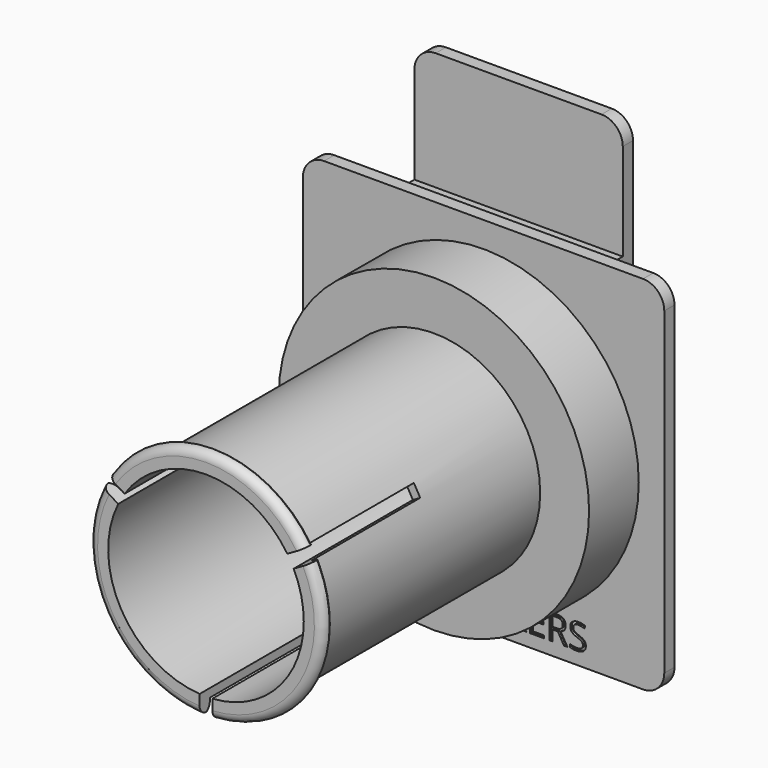
from build123d import *

# Parameters (mm, degrees)
F3_DEPTH      = 3
F4_W          = 49
F4_H          = 3
F5_DEPTH      = 7.3
F7_DEPTH      = 3
F8_R          = 36.5
F9_DEPTH      = 14.6
F10_R         = 25
F11_DEPTH     = 64
F12_R         = 23
F13_DEPTH     = 81.6
F14_R         = 27.5
F14_R_2       = 23
F15_DEPTH     = 3
F17_DEPTH     = 35
F18_R         = 2
F19_T2_ANGLE  = 95.8983460489
F19_T4_ANGLE  = 131.8015185297
F19_T6_ANGLE  = 131.8015185297
F19_T8_ANGLE  = 35.8952924791
F20_TEXT_SIZE = 8.3333333333
F21_DEPTH     = 0.5


# Not quite as in the source:
# - a fillet or chamfer that OpenCascade refuses, or shapes differently, is made with other operations: its cross-section is extruded or revolved along the edge and cut away or added
# - a feature names something its author has since deleted; it is built from what else it names
# - Text() gives the source's letters only with a copy of the font that has no kerning and outlines rounded to 1/6400 em; it was checked with that copy


with BuildPart() as f3:
    # F2 (on Front) → F3 (new body)
    with BuildSketch(Plane.XZ):
        with BuildLine():
            Line((-5, 38.3), (-44, 38.3))
            ThreePointArc((-44, 38.3), (-47.5355339059, 36.8355339059), (-49, 33.3))
            Line((-49, 33.3), (-49, 5))
            ThreePointArc((-49, 5), (-47.5355339059, 1.4644660941), (-44, 0))
            Line((-44, 0), (-5, 0))
            ThreePointArc((-5, 0), (-1.4644660941, 1.4644660941), (0, 5))
            Line((0, 5), (0, 33.3))
            ThreePointArc((0, 33.3), (-1.4644660941, 36.8355339059), (-5, 38.3))
        make_face()
    extrude(amount=F3_DEPTH)

    # F4 (on face) → F5 (join)
    with BuildSketch(Plane.XZ.offset(3)):
        with Locations((-24.5, 9)):
            Rectangle(F4_W, F4_H)
    extrude(amount=F5_DEPTH)

    # F6 (on face) → F7 (join)
    with BuildSketch(Plane.XZ.offset(10.3)):
        with BuildLine():
            Line((13, 14.3), (-62, 14.3))
            ThreePointArc((-62, 14.3), (-65.5355339059, 12.8355339059), (-67, 9.3))
            Line((-67, 9.3), (-67, -65.7))
            ThreePointArc((-67, -65.7), (-65.5355339059, -69.2355339059), (-62, -70.7))
            Line((-62, -70.7), (13, -70.7))
            ThreePointArc((13, -70.7), (16.5355339059, -69.2355339059), (18, -65.7))
            Line((18, -65.7), (18, 9.3))
            ThreePointArc((18, 9.3), (16.5355339059, 12.8355339059), (13, 14.3))
        make_face()
    extrude(amount=F7_DEPTH)

    # F8 (on face) → F9 (join)
    with BuildSketch(Plane.XZ.offset(13.3)):
        with Locations((-24.5, -28.2)):
            Circle(F8_R)
    extrude(amount=F9_DEPTH)

    # F10 (on face) → F11 (join)
    with BuildSketch(Plane.XZ.offset(27.9)):
        with Locations((-24.5, -28.2)):
            Circle(F10_R)
    extrude(amount=F11_DEPTH)

    # F12 (on face) → F13 (cut, through all)
    with BuildSketch(Plane.XZ.offset(91.9)):
        with Locations((-24.5, -28.2)):
            Circle(F12_R)
    extrude(amount=-F13_DEPTH, mode=Mode.SUBTRACT)

    # F14 (on face) → F15 (join)
    with BuildSketch(Plane.XZ.offset(91.9)):
        with Locations((-24.5, -28.2)):
            Circle(F14_R)
        with Locations((-24.5, -28.2)):
            Circle(F14_R_2, mode=Mode.SUBTRACT)
    extrude(amount=F15_DEPTH)

    # F16 (on face) → F17 (cut, symmetric)
    with BuildSketch(Plane.XZ.offset(94.9)):
        Polygon((-26, -29.0660254038), (-26, -28.2), (-24.5, -28.2), (-25.25, -26.9009618943), (-24.5, -26.4679491924), (-50.2167782531, -11.6203603453), (-51.7167782531, -14.2184365567), align=None)
        Polygon((-24.5, -28.2), (-26, -28.2), (-26, -29.0660254038), (-25.25, -29.4990381057), align=None)
        Polygon((-23.75, -26.9009618943), (-24.5, -28.2), (-23, -28.2), (-23, -29.0660254038), (2.7167782531, -14.2184365567), (1.2167782531, -11.6203603453), (-24.5, -26.4679491924), align=None)
        Polygon((-23, -28.2), (-24.5, -28.2), (-23.75, -29.4990381057), (-23, -29.0660254038), align=None)
        Polygon((-23.75, -29.4990381057), (-24.5, -28.2), (-25.25, -29.4990381057), (-26, -29.0660254038), (-26, -58.761203098), (-23, -58.761203098), (-23, -29.0660254038), align=None)
        Polygon((-25.25, -26.9009618943), (-24.5, -28.2), (-23.75, -26.9009618943), (-24.5, -26.4679491924), align=None)
    extrude(amount=F17_DEPTH, both=True, mode=Mode.SUBTRACT)

    # F18
    f18_edges = [f3.edges().sort_by_distance(p)[0] for p in [
        (-48.315699, -94.9, -41.95),
        (-24.5, -94.9, -0.7),
        (-4.531274, -94.9, -47.10767),
    ]]
    fillet(f18_edges, radius=F18_R)

    # F19: fillet of radius 2 on 3 edges, made by hand

    # F19_s1 → F19_t2 (revolve, cut)
    with BuildSketch(Plane(origin=(-21.3586726372, 0, 2.2065809656), x_dir=(0, 1, 0), z_dir=(-0.994705784, 0, 0.1027638228))):
        with BuildLine():
            ThreePointArc((-91.9, 56.3363659591), (-92.1679491924, 57.3363659591), (-92.9, 58.0684167666))
            Line((-92.9, 58.0684167666), (-91.9, 58.0684167666))
            Line((-91.9, 58.0684167666), (-91.9, 56.3363659591))
        make_face()
    revolve(axis=Axis((-24.5, -91.9, -28.2), (0, -1, 0)), revolution_arc=F19_T2_ANGLE, mode=Mode.SUBTRACT)

    # F19_s3 → F19_t4 (revolve, cut)
    with BuildSketch(Plane(origin=(6.4262272989, 0, -14.366521817), x_dir=(0, 1, 0), z_dir=(0.4083183638, 0, -0.9128395882))):
        with BuildLine():
            ThreePointArc((-91.9, -8.111198577), (-92.1679491924, -7.111198577), (-92.9, -6.3791477695))
            Line((-92.9, -6.3791477695), (-91.9, -6.3791477695))
            Line((-91.9, -6.3791477695), (-91.9, -8.111198577))
        make_face()
    revolve(axis=Axis((-24.5, -91.9, -28.2), (0, -1, 0)), revolution_arc=F19_T4_ANGLE, mode=Mode.SUBTRACT)

    # F19_s5 → F19_t6 (revolve, cut)
    with BuildSketch(Plane(origin=(-21.8189283136, 0, -30.1408263792), x_dir=(0, 1, 0), z_dir=(0.5863830911, 0, 0.81003387))):
        with BuildLine():
            ThreePointArc((-91.9, 29.0777758377), (-92.1679491924, 30.0777758377), (-92.9, 30.8098266453))
            Line((-92.9, 30.8098266453), (-91.9, 30.8098266453))
            Line((-91.9, 30.8098266453), (-91.9, 29.0777758377))
        make_face()
    revolve(axis=Axis((-24.5, -91.9, -28.2), (0, -1, 0)), revolution_arc=F19_T6_ANGLE, mode=Mode.SUBTRACT)

    # F19_s7 → F19_t8 (revolve, cut)
    with BuildSketch(Plane.XY.offset(-28.2)):
        with BuildLine():
            ThreePointArc((3, -92.9), (2.2679491924, -92.1679491924), (1.2679491924, -91.9))
            Line((1.2679491924, -91.9), (3, -91.9))
            Line((3, -91.9), (3, -92.9))
        make_face()
    revolve(axis=Axis((-24.5, -91.9, -28.2), (0, -1, 0)), revolution_arc=F19_T8_ANGLE, mode=Mode.SUBTRACT)

    # F20 (on face) → F21 (cut)
    with BuildSketch(Plane.XZ.offset(13.3)):
        with Locations((-49.099609375, -67.7)):
            Text('DIGIMAKERS', F20_TEXT_SIZE, font='Open Sans', text_align=(TextAlign.LEFT, TextAlign.BOTTOM))
    extrude(amount=-F21_DEPTH, mode=Mode.SUBTRACT)


solid = f3.part
